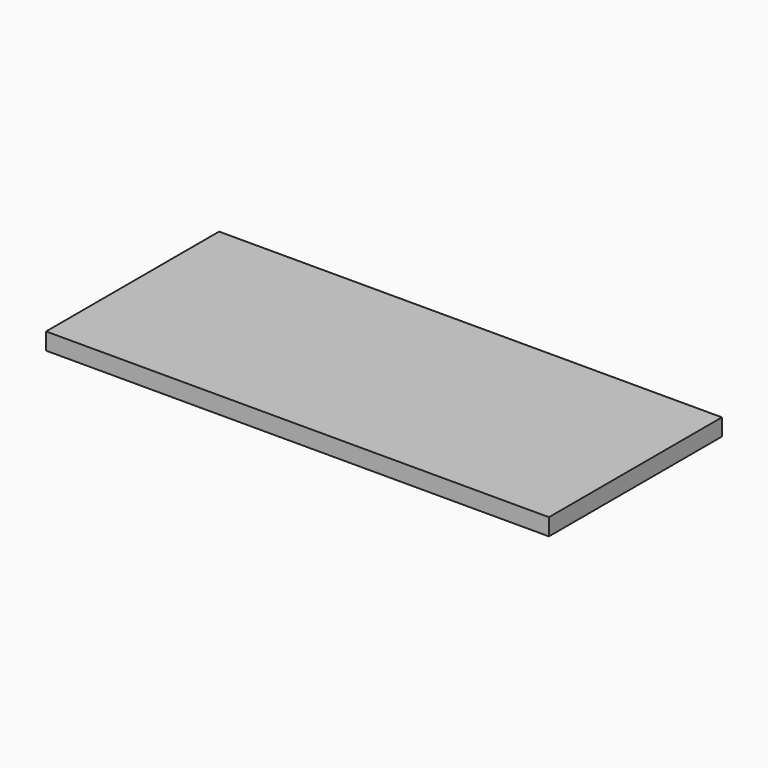
from build123d import *

# Parameters (mm, degrees)
F2_DEPTH     = 1.27
F0_TEXT_SIZE = 3.175
F3_DEPTH     = 1.1938


# Not quite as in the source:
# - Text() gives the source's letters only with a copy of the font that has no kerning and outlines rounded to 1/6400 em; it was checked with that copy


with BuildPart() as f2:
    # F1 (on Top) → F2 (new body)
    with BuildSketch(Plane.XY):
        Polygon((-1.5709077707, 0), (0, 0), (36.1005365849, 0), (36.1005365849, 16.1986146122), (-1.5709077707, 16.1986146122), align=None)
    extrude(amount=F2_DEPTH)

    # F0 (on Top) → F3 (join)
    with BuildSketch(Plane.XY):
        with Locations((1.1576538767, 11.3797230955)):
            Text('This is just the start.', F0_TEXT_SIZE, font='Tinos', text_align=(TextAlign.LEFT, TextAlign.BOTTOM))
        with Locations((1.1576538767, 7.7284730955)):
            Text('Nails to heart ventricle:', F0_TEXT_SIZE, font='Tinos', text_align=(TextAlign.LEFT, TextAlign.BOTTOM))
        with Locations((1.1576538767, 4.0772230955)):
            Text('I will fall apart.', F0_TEXT_SIZE, font='Tinos', text_align=(TextAlign.LEFT, TextAlign.BOTTOM))
    extrude(amount=-F3_DEPTH)


solid = f2.part
